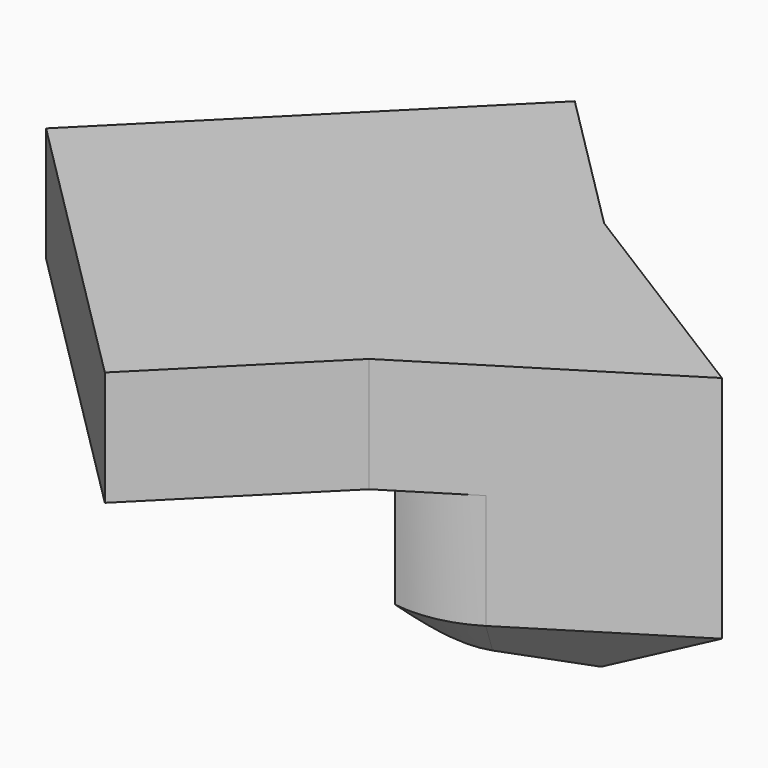
from build123d import *

# Parameters (mm, degrees)
F1_W         = 18.1
F1_H         = 18.1
F2_DEPTH     = 5
F3_W         = 16.1
F3_H         = 16.1
F4_DEPTH     = 4
F5_ANGLE     = 45
F7_DEPTH     = 5
F9_DEPTH     = 8
F10_T1_DEPTH = 17.995241473
F11_T1_DEPTH = 15.801577482
F11_T3_DEPTH = 15.801577482
F11_T6_ANGLE = 128.9448568851
F11_T8_ANGLE = 128.9448568851


# Not quite as in the source:
# - a fillet or chamfer that OpenCascade refuses, or shapes differently, is made with other operations: its cross-section is extruded or revolved along the edge and cut away or added


with BuildPart() as f2:
    # F1 (on Top) → F2 (new body)
    with BuildSketch(Plane.XY):
        Rectangle(F1_W, F1_H)
    extrude(amount=F2_DEPTH)

    # F3 (on Top) → F4 (cut)
    with BuildSketch(Plane.XY):
        Rectangle(F3_W, F3_H)
    extrude(amount=F4_DEPTH, mode=Mode.SUBTRACT)


with BuildPart() as f2_1:
    # F5: moved
    add(f2.part.rotate(Axis((0, 0, 23.8891355693), (0, 0, 1)), F5_ANGLE))

    # F6 (on face) → F7 (join)
    with BuildSketch(Plane.XY.offset(5)):
        Polygon((12.7986327395, 0), (6.3993163697, -6.3993163697), (16.6505072266, 0), (6.3993163697, 6.3993163697), align=None)
    extrude(amount=-F7_DEPTH)

    # F8 (on face) → F9 (join)
    with BuildSketch(Plane(origin=(0, 0, 0), x_dir=(1, 0, 0), z_dir=(0, 0, -1))):
        Polygon((16.6505072266, 0), (6.3993163697, 6.3993163697), (6.3993163697, 4.9851028074), (11.3844191771, 0), (6.3993163697, -4.9851028074), (6.3993163697, -6.3993163697), align=None)
    extrude(amount=F9_DEPTH)

    # F10: fillet of radius 5 on 2 edges, made by hand

    # F10_s2 → F10_t1 (cut)
    with BuildSketch(Plane.XY.offset(-17.995241473)):
        with BuildLine():
            ThreePointArc((6.3993163697, -4.9851028074), (8.1578886795, -4.9366807501), (9.7908366557, -4.2821563649))
            Line((9.7908366557, -4.2821563649), (6.3993163697, -6.3993163697))
            Line((6.3993163697, -6.3993163697), (6.3993163697, -4.9851028074))
        make_face()
        with BuildLine():
            ThreePointArc((9.7908366557, 4.2821563649), (8.1578886795, 4.9366807501), (6.3993163697, 4.9851028074))
            Line((6.3993163697, 4.9851028074), (6.3993163697, 6.3993163697))
            Line((6.3993163697, 6.3993163697), (9.7908366557, 4.2821563649))
        make_face()
    extrude(amount=F10_T1_DEPTH, mode=Mode.SUBTRACT)

    # F11: chamfer of 3 on 2 edges, made by hand

    # F11_s2 → F11_t1 (cut)
    with BuildSketch(Plane(origin=(5.1217894323, -3.1972822879, 0), x_dir=(0, 0, 1), z_dir=(0.8482837296, -0.5295419852, 0))):
        Polygon((-5, -8.8171426514), (-8, -5.8171426514), (-8, -8.8171426514), align=None)
    extrude(amount=F11_T1_DEPTH, mode=Mode.SUBTRACT)

    # F11_s4 → F11_t3 (cut)
    with BuildSketch(Plane(origin=(18.5260105123, 11.564880997, 0), x_dir=(0, 0, 1), z_dir=(-0.8482837296, -0.5295419852, 0))):
        Polygon((-5, -8.8171426514), (-8, -5.8171426514), (-8, -8.8171426514), align=None)
    extrude(amount=F11_T3_DEPTH, mode=Mode.SUBTRACT)

    # F11_s5 → F11_t6 (revolve, cut)
    with BuildSketch(Plane(origin=(5.1217894331, 3.1972822878, 0), x_dir=(0, 0, 1), z_dir=(0.8482837296, 0.5295419851, 0))):
        Polygon((-8, 5.8171426509), (-5, 8.8171426509), (-8, 8.8171426509), align=None)
    revolve(axis=Axis((7.1431267295, -0.0407377158, -8), (0, 0, -1)), revolution_arc=F11_T6_ANGLE, mode=Mode.SUBTRACT)

    # F11_s7 → F11_t8 (revolve, cut)
    with BuildSketch(Plane(origin=(0.1002908696, -0.8203136168, 0), x_dir=(0, 0, 1), z_dir=(0.1213555739, -0.9926090996, 0))):
        Polygon((-8, -5.0952763393), (-5, -2.0952763393), (-8, -2.0952763393), align=None)
    revolve(axis=Axis((7.1431267295, 0.0407377158, -8), (0, 0, -1)), revolution_arc=F11_T8_ANGLE, mode=Mode.SUBTRACT)


solid = f2_1.part
